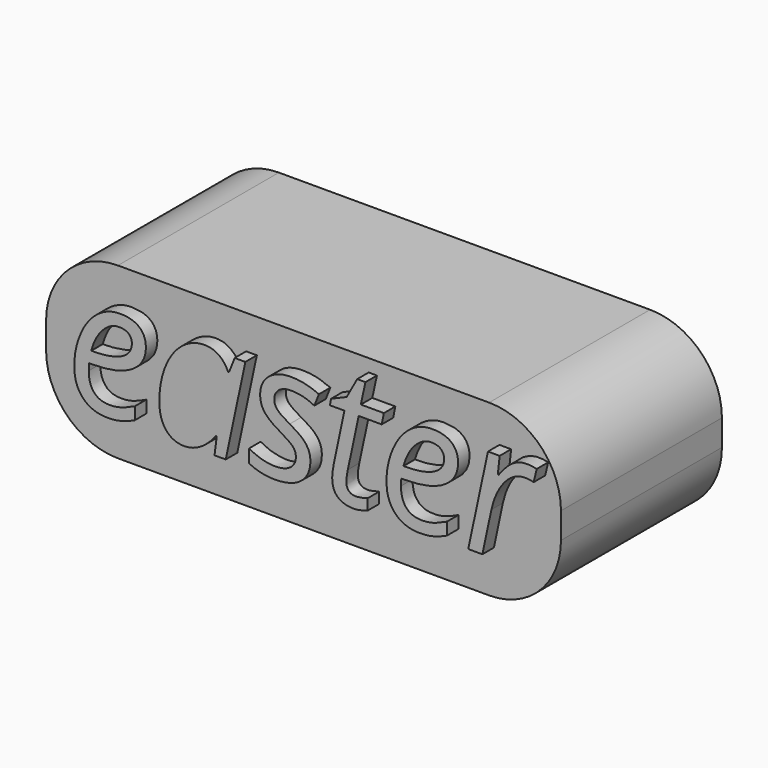
from build123d import *

# Parameters (mm, degrees)
F0_TEXT_SIZE = 12.0000000751
F1_DEPTH     = 15
F3_DEPTH     = 14


# Not quite as in the source:
# - Text() gives the source's letters only with a copy of the font that has no kerning and outlines rounded to 1/6400 em; it was checked with that copy


with BuildPart() as f1:
    # F0 (on Front) → F1 (new body)
    with BuildSketch(Plane.XZ):
        with Locations((-16.7999994223, -3.872000739)):
            Text('easter', F0_TEXT_SIZE, font='Open Sans', font_style=FontStyle.ITALIC, text_align=(TextAlign.LEFT, TextAlign.BOTTOM))
        with BuildLine():
            add(Edge.make_bspline(
                [(-9.0243743736, -2.8435632325), (-8.7487493719, -3.1745007346), (-8.2518743688, -3.1745007346)],
                knots=[0, 0, 0, 1, 1, 1], degree=2))
            add(Edge.make_bspline(
                [(-8.2518743688, -3.1745007346), (-7.6837493652, -3.1745007346), (-7.1212493617, -2.6326257312)],
                knots=[0, 0, 0, 1, 1, 1], degree=2))
            add(Edge.make_bspline(
                [(-7.1212493617, -2.6326257312), (-6.5587493582, -2.0907507278), (-6.207186856, -1.2207507224)],
                knots=[0, 0, 0, 1, 1, 1], degree=2))
            add(Edge.make_bspline(
                [(-6.207186856, -1.2207507224), (-5.8556243538, -0.3507507169), (-5.8556243538, 0.5229992885)],
                knots=[0, 0, 0, 1, 1, 1], degree=2))
            add(Edge.make_bspline(
                [(-5.8556243538, 0.5229992885), (-5.8556243538, 1.1267492923), (-6.1837493558, 1.4839367945)],
                knots=[0, 0, 0, 1, 1, 1], degree=2))
            add(Edge.make_bspline(
                [(-6.1837493558, 1.4839367945), (-6.5118743579, 1.8411242968), (-7.0443743612, 1.8411242968)],
                knots=[0, 0, 0, 1, 1, 1], degree=2))
            add(Edge.make_bspline(
                [(-7.0443743612, 1.8411242968), (-7.653749365, 1.8411242968), (-8.1778118683, 1.3367492936)],
                knots=[0, 0, 0, 1, 1, 1], degree=2))
            add(Edge.make_bspline(
                [(-8.1778118683, 1.3367492936), (-8.7018743716, 0.8323742905), (-9.0009368735, -0.0282507149)],
                knots=[0, 0, 0, 1, 1, 1], degree=2))
            add(Edge.make_bspline(
                [(-9.0009368735, -0.0282507149), (-9.2999993753, -0.8888757203), (-9.2999993753, -1.8451257263)],
                knots=[0, 0, 0, 1, 1, 1], degree=2))
            add(Edge.make_bspline(
                [(-9.2999993753, -1.8451257263), (-9.2999993753, -2.5126257305), (-9.0243743736, -2.8435632325)],
                knots=[0, 0, 0, 1, 1, 1], degree=2))
        make_face()
    extrude(amount=F1_DEPTH)


with BuildPart() as f3:
    # F2 (on Front) → F3 (new body)
    with BuildSketch(Plane.XZ):
        with BuildLine():
            Line((11.8447784628, 4.9076448301), (-13.9877492717, 4.9076448301))
            ThreePointArc((-13.9877492717, 4.9076448301), (-17.5232831776, 3.4431787361), (-18.9877492717, -0.0923551699))
            Line((-18.9877492717, -0.0923551699), (-18.9877492717, -1.9067989314))
            ThreePointArc((-18.9877492717, -1.9067989314), (-17.5232831776, -5.4423328374), (-13.9877492717, -6.9067989314))
            Line((-13.9877492717, -6.9067989314), (11.8447784628, -6.9067989314))
            ThreePointArc((11.8447784628, -6.9067989314), (15.3803123687, -5.4423328374), (16.8447784628, -1.9067989314))
            Line((16.8447784628, -1.9067989314), (16.8447784628, -0.0923551699))
            ThreePointArc((16.8447784628, -0.0923551699), (15.3803123687, 3.4431787361), (11.8447784628, 4.9076448301))
        make_face()
    extrude(amount=F3_DEPTH)


solid = Compound([f1.part, f3.part])
